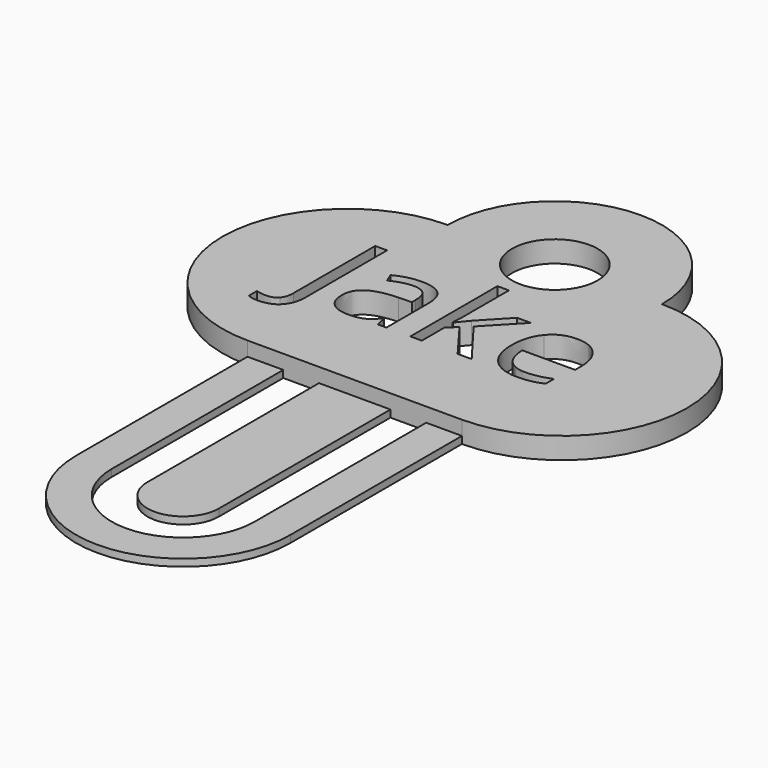
from build123d import *

# Parameters (mm, degrees)
F0_R     = 6
F1_DEPTH = 3
F2_DEPTH = 1


with BuildPart() as f1:
    # F0 (on Top) → F1 (new body)
    with BuildSketch(Plane.XY):
        with BuildLine():
            Line((10, -17.5), (15, -17.5))
            ThreePointArc((15, -17.5), (32.5, 0), (15, 17.5))
            ThreePointArc((15, 17.5), (0, 32.5), (-15, 17.5))
            ThreePointArc((-15, 17.5), (-32.5, 0), (-15, -17.5))
            Line((-15, -17.5), (-10, -17.5))
            Line((-10, -17.5), (-5, -17.5))
            Line((-5, -17.5), (5, -17.5))
            Line((5, -17.5), (10, -17.5))
        make_face()
        with BuildLine():
            add(Edge.make_bspline(
                [(-17.3530564989, -8.385057961), (-18.2929470593, -9.4079721875), (-20.0568083443, -9.4079721875)],
                knots=[0, 0, 0, 1, 1, 1], degree=2))
            add(Edge.make_bspline(
                [(-20.0568083443, -9.4079721875), (-20.974768125, -9.4079721875), (-21.5042398074, -9.1448028306)],
                knots=[0, 0, 0, 1, 1, 1], degree=2))
            Line((-21.5042398074, -9.1448028306), (-21.5042398074, -7.7255680844))
            add(Edge.make_bspline(
                [(-21.5042398074, -7.7255680844), (-20.8087207927, -7.9198121336), (-20.0568083443, -7.9198121336)],
                knots=[0, 0, 0, 1, 1, 1], degree=2))
            add(Edge.make_bspline(
                [(-20.0568083443, -7.9198121336), (-19.0855880986, -7.9198121336), (-18.5811801645, -7.3323805333)],
                knots=[0, 0, 0, 1, 1, 1], degree=2))
            add(Edge.make_bspline(
                [(-18.5811801645, -7.3323805333), (-18.0767722304, -6.7449489331), (-18.0767722304, -5.6390110403)],
                knots=[0, 0, 0, 1, 1, 1], degree=2))
            Line((-18.0767722304, -5.6390110403), (-18.0767722304, 8.6755221946))
            Line((-18.0767722304, 8.6755221946), (-16.4131659385, 8.6755221946))
            Line((-16.4131659385, 8.6755221946), (-16.4131659385, -5.5011604248))
            add(Edge.make_bspline(
                [(-16.4131659385, -5.5011604248), (-16.4131659385, -7.3621437344), (-17.3530564989, -8.385057961)],
                knots=[0, 0, 0, 1, 1, 1], degree=2))
        make_face(mode=Mode.SUBTRACT)
        with BuildLine():
            Line((-5.0561550003, -5.6390110403), (-6.2623478861, -5.6390110403))
            Line((-6.2623478861, -5.6390110403), (-6.5850436452, -4.1101223954))
            Line((-6.5850436452, -4.1101223954), (-6.6633678586, -4.1101223954))
            add(Edge.make_bspline(
                [(-6.6633678586, -4.1101223954), (-7.4654078035, -5.1189382636), (-8.2627482955, -5.4776631608)],
                knots=[0, 0, 0, 1, 1, 1], degree=2))
            add(Edge.make_bspline(
                [(-8.2627482955, -5.4776631608), (-9.0600887876, -5.836388058), (-10.2568827679, -5.836388058)],
                knots=[0, 0, 0, 1, 1, 1], degree=2))
            add(Edge.make_bspline(
                [(-10.2568827679, -5.836388058), (-11.851563752, -5.836388058), (-12.7569916585, -5.0124173334)],
                knots=[0, 0, 0, 1, 1, 1], degree=2))
            add(Edge.make_bspline(
                [(-12.7569916585, -5.0124173334), (-13.6624195651, -4.1884466088), (-13.6624195651, -2.672089838)],
                knots=[0, 0, 0, 1, 1, 1], degree=2))
            add(Edge.make_bspline(
                [(-13.6624195651, -2.672089838), (-13.6624195651, 0.5767985325), (-8.464824766, 0.7334469592)],
                knots=[0, 0, 0, 1, 1, 1], degree=2))
            Line((-8.464824766, 0.7334469592), (-6.6445700474, 0.7929733614))
            Line((-6.6445700474, 0.7929733614), (-6.6445700474, 1.4602956592))
            add(Edge.make_bspline(
                [(-6.6445700474, 1.4602956592), (-6.6445700474, 2.7228819787), (-7.1865736039, 3.3244119374)],
                knots=[0, 0, 0, 1, 1, 1], degree=2))
            add(Edge.make_bspline(
                [(-7.1865736039, 3.3244119374), (-7.7285771604, 3.925941896), (-8.9253711406, 3.925941896)],
                knots=[0, 0, 0, 1, 1, 1], degree=2))
            add(Edge.make_bspline(
                [(-8.9253711406, 3.925941896), (-10.2662816735, 3.925941896), (-11.9580846822, 3.10510414)],
                knots=[0, 0, 0, 1, 1, 1], degree=2))
            Line((-11.9580846822, 3.10510414), (-12.4593596477, 4.3488926482))
            add(Edge.make_bspline(
                [(-12.4593596477, 4.3488926482), (-11.6667186085, 4.7781093375), (-10.7221285953, 5.0224808832)],
                knots=[0, 0, 0, 1, 1, 1], degree=2))
            add(Edge.make_bspline(
                [(-10.7221285953, 5.0224808832), (-9.7775385821, 5.2668524289), (-8.8251161475, 5.2668524289)],
                knots=[0, 0, 0, 1, 1, 1], degree=2))
            add(Edge.make_bspline(
                [(-8.8251161475, 5.2668524289), (-6.9077394043, 5.2668524289), (-5.9819472023, 4.4162514717)],
                knots=[0, 0, 0, 1, 1, 1], degree=2))
            add(Edge.make_bspline(
                [(-5.9819472023, 4.4162514717), (-5.0561550003, 3.5656505146), (-5.0561550003, 1.6858693937)],
                knots=[0, 0, 0, 1, 1, 1], degree=2))
            Line((-5.0561550003, 1.6858693937), (-5.0561550003, -5.6390110403))
        make_face(mode=Mode.SUBTRACT)
        with BuildLine():
            Line((-0.1812559603, -0.146917199), (-0.102931747, -0.146917199))
            add(Edge.make_bspline(
                [(-0.102931747, -0.146917199), (0.3168860367, 0.4514797911), (1.1784523837, 1.4195670683)],
                knots=[0, 0, 0, 1, 1, 1], degree=2))
            Line((1.1784523837, 1.4195670683), (4.6435155831, 5.0914061909))
            Line((4.6435155831, 5.0914061909), (6.5734242004, 5.0914061909))
            Line((6.5734242004, 5.0914061909), (2.2248638743, 0.5204050988))
            Line((2.2248638743, 0.5204050988), (6.8773221483, -5.6390110403))
            Line((6.8773221483, -5.6390110403), (4.9098179085, -5.6390110403))
            Line((4.9098179085, -5.6390110403), (1.1189259815, -0.5667349827))
            Line((1.1189259815, -0.5667349827), (-0.102931747, -1.6256783474))
            Line((-0.102931747, -1.6256783474), (-0.102931747, -5.6390110403))
            Line((-0.102931747, -5.6390110403), (-1.7101446053, -5.6390110403))
            Line((-1.7101446053, -5.6390110403), (-1.7101446053, 9.5966149438))
            Line((-1.7101446053, 9.5966149438), (-0.102931747, 9.5966149438))
            Line((-0.102931747, 9.5966149438), (-0.102931747, 1.5166890929))
            add(Edge.make_bspline(
                [(-0.102931747, 1.5166890929), (-0.102931747, 0.9809514734), (-0.1812559603, -0.146917199)],
                knots=[0, 0, 0, 1, 1, 1], degree=2))
        make_face(mode=Mode.SUBTRACT)
        with BuildLine():
            add(Edge.make_bspline(
                [(15.2016195449, -5.6734736942), (14.4340422539, -5.836388058), (13.3469021724, -5.836388058)],
                knots=[0, 0, 0, 1, 1, 1], degree=2))
            add(Edge.make_bspline(
                [(13.3469021724, -5.836388058), (10.9689790546, -5.836388058), (9.5920393836, -4.3858236265)],
                knots=[0, 0, 0, 1, 1, 1], degree=2))
            add(Edge.make_bspline(
                [(9.5920393836, -4.3858236265), (8.2150997126, -2.9352591949), (8.2150997126, -0.3630920279)],
                knots=[0, 0, 0, 1, 1, 1], degree=2))
            add(Edge.make_bspline(
                [(8.2150997126, -0.3630920279), (8.2150997126, 2.2341388873), (9.4933508747, 3.761461048)],
                knots=[0, 0, 0, 1, 1, 1], degree=2))
            add(Edge.make_bspline(
                [(9.4933508747, 3.761461048), (10.7716020369, 5.2887832086), (12.9270843887, 5.2887832086)],
                knots=[0, 0, 0, 1, 1, 1], degree=2))
            add(Edge.make_bspline(
                [(12.9270843887, 5.2887832086), (14.9415831565, 5.2887832086), (16.116446357, 3.9619710342)],
                knots=[0, 0, 0, 1, 1, 1], degree=2))
            add(Edge.make_bspline(
                [(16.116446357, 3.9619710342), (17.2913095575, 2.6351588598), (17.2913095575, 0.4608786967)],
                knots=[0, 0, 0, 1, 1, 1], degree=2))
            Line((17.2913095575, 0.4608786967), (17.2913095575, -0.5667349827))
            Line((17.2913095575, -0.5667349827), (9.9006367842, -0.5667349827))
            add(Edge.make_bspline(
                [(9.9006367842, -0.5667349827), (9.9507642808, -2.4559150091), (10.8561921873, -3.4349676762)],
                knots=[0, 0, 0, 1, 1, 1], degree=2))
            add(Edge.make_bspline(
                [(10.8561921873, -3.4349676762), (11.7616200938, -4.4140203433), (13.4064285746, -4.4140203433)],
                knots=[0, 0, 0, 1, 1, 1], degree=2))
            add(Edge.make_bspline(
                [(13.4064285746, -4.4140203433), (15.1389601742, -4.4140203433), (16.830763183, -3.6903046118)],
                knots=[0, 0, 0, 1, 1, 1], degree=2))
            Line((16.830763183, -3.6903046118), (16.830763183, -5.1408690433))
            add(Edge.make_bspline(
                [(16.830763183, -5.1408690433), (15.9691968359, -5.5105593304), (15.2016195449, -5.6734736942)],
                knots=[0, 0, 0, 1, 1, 1], degree=2))
        make_face(mode=Mode.SUBTRACT)
        with Locations((0, 17.5)):
            Circle(F0_R, mode=Mode.SUBTRACT)
    extrude(amount=F1_DEPTH)

    # F0 (on Top) → F2 (join)
    with BuildSketch(Plane.XY):
        with BuildLine():
            Line((15, -47.5), (15, -17.5))
            Line((15, -17.5), (10, -17.5))
            Line((10, -17.5), (10, -47.5))
            ThreePointArc((10, -47.5), (0, -57.5), (-10, -47.5))
            Line((-10, -47.5), (-10, -17.5))
            Line((-10, -17.5), (-15, -17.5))
            Line((-15, -17.5), (-15, -47.5))
            ThreePointArc((-15, -47.5), (0, -62.5), (15, -47.5))
        make_face()
        with BuildLine():
            Line((10, -17.5), (15, -17.5))
            ThreePointArc((15, -17.5), (32.5, 0), (15, 17.5))
            ThreePointArc((15, 17.5), (0, 32.5), (-15, 17.5))
            ThreePointArc((-15, 17.5), (-32.5, 0), (-15, -17.5))
            Line((-15, -17.5), (-10, -17.5))
            Line((-10, -17.5), (-5, -17.5))
            Line((-5, -17.5), (5, -17.5))
            Line((5, -17.5), (10, -17.5))
        make_face()
        with BuildLine():
            add(Edge.make_bspline(
                [(-17.3530564989, -8.385057961), (-18.2929470593, -9.4079721875), (-20.0568083443, -9.4079721875)],
                knots=[0, 0, 0, 1, 1, 1], degree=2))
            add(Edge.make_bspline(
                [(-20.0568083443, -9.4079721875), (-20.974768125, -9.4079721875), (-21.5042398074, -9.1448028306)],
                knots=[0, 0, 0, 1, 1, 1], degree=2))
            Line((-21.5042398074, -9.1448028306), (-21.5042398074, -7.7255680844))
            add(Edge.make_bspline(
                [(-21.5042398074, -7.7255680844), (-20.8087207927, -7.9198121336), (-20.0568083443, -7.9198121336)],
                knots=[0, 0, 0, 1, 1, 1], degree=2))
            add(Edge.make_bspline(
                [(-20.0568083443, -7.9198121336), (-19.0855880986, -7.9198121336), (-18.5811801645, -7.3323805333)],
                knots=[0, 0, 0, 1, 1, 1], degree=2))
            add(Edge.make_bspline(
                [(-18.5811801645, -7.3323805333), (-18.0767722304, -6.7449489331), (-18.0767722304, -5.6390110403)],
                knots=[0, 0, 0, 1, 1, 1], degree=2))
            Line((-18.0767722304, -5.6390110403), (-18.0767722304, 8.6755221946))
            Line((-18.0767722304, 8.6755221946), (-16.4131659385, 8.6755221946))
            Line((-16.4131659385, 8.6755221946), (-16.4131659385, -5.5011604248))
            add(Edge.make_bspline(
                [(-16.4131659385, -5.5011604248), (-16.4131659385, -7.3621437344), (-17.3530564989, -8.385057961)],
                knots=[0, 0, 0, 1, 1, 1], degree=2))
        make_face(mode=Mode.SUBTRACT)
        with BuildLine():
            Line((-5.0561550003, -5.6390110403), (-6.2623478861, -5.6390110403))
            Line((-6.2623478861, -5.6390110403), (-6.5850436452, -4.1101223954))
            Line((-6.5850436452, -4.1101223954), (-6.6633678586, -4.1101223954))
            add(Edge.make_bspline(
                [(-6.6633678586, -4.1101223954), (-7.4654078035, -5.1189382636), (-8.2627482955, -5.4776631608)],
                knots=[0, 0, 0, 1, 1, 1], degree=2))
            add(Edge.make_bspline(
                [(-8.2627482955, -5.4776631608), (-9.0600887876, -5.836388058), (-10.2568827679, -5.836388058)],
                knots=[0, 0, 0, 1, 1, 1], degree=2))
            add(Edge.make_bspline(
                [(-10.2568827679, -5.836388058), (-11.851563752, -5.836388058), (-12.7569916585, -5.0124173334)],
                knots=[0, 0, 0, 1, 1, 1], degree=2))
            add(Edge.make_bspline(
                [(-12.7569916585, -5.0124173334), (-13.6624195651, -4.1884466088), (-13.6624195651, -2.672089838)],
                knots=[0, 0, 0, 1, 1, 1], degree=2))
            add(Edge.make_bspline(
                [(-13.6624195651, -2.672089838), (-13.6624195651, 0.5767985325), (-8.464824766, 0.7334469592)],
                knots=[0, 0, 0, 1, 1, 1], degree=2))
            Line((-8.464824766, 0.7334469592), (-6.6445700474, 0.7929733614))
            Line((-6.6445700474, 0.7929733614), (-6.6445700474, 1.4602956592))
            add(Edge.make_bspline(
                [(-6.6445700474, 1.4602956592), (-6.6445700474, 2.7228819787), (-7.1865736039, 3.3244119374)],
                knots=[0, 0, 0, 1, 1, 1], degree=2))
            add(Edge.make_bspline(
                [(-7.1865736039, 3.3244119374), (-7.7285771604, 3.925941896), (-8.9253711406, 3.925941896)],
                knots=[0, 0, 0, 1, 1, 1], degree=2))
            add(Edge.make_bspline(
                [(-8.9253711406, 3.925941896), (-10.2662816735, 3.925941896), (-11.9580846822, 3.10510414)],
                knots=[0, 0, 0, 1, 1, 1], degree=2))
            Line((-11.9580846822, 3.10510414), (-12.4593596477, 4.3488926482))
            add(Edge.make_bspline(
                [(-12.4593596477, 4.3488926482), (-11.6667186085, 4.7781093375), (-10.7221285953, 5.0224808832)],
                knots=[0, 0, 0, 1, 1, 1], degree=2))
            add(Edge.make_bspline(
                [(-10.7221285953, 5.0224808832), (-9.7775385821, 5.2668524289), (-8.8251161475, 5.2668524289)],
                knots=[0, 0, 0, 1, 1, 1], degree=2))
            add(Edge.make_bspline(
                [(-8.8251161475, 5.2668524289), (-6.9077394043, 5.2668524289), (-5.9819472023, 4.4162514717)],
                knots=[0, 0, 0, 1, 1, 1], degree=2))
            add(Edge.make_bspline(
                [(-5.9819472023, 4.4162514717), (-5.0561550003, 3.5656505146), (-5.0561550003, 1.6858693937)],
                knots=[0, 0, 0, 1, 1, 1], degree=2))
            Line((-5.0561550003, 1.6858693937), (-5.0561550003, -5.6390110403))
        make_face(mode=Mode.SUBTRACT)
        with BuildLine():
            Line((-0.1812559603, -0.146917199), (-0.102931747, -0.146917199))
            add(Edge.make_bspline(
                [(-0.102931747, -0.146917199), (0.3168860367, 0.4514797911), (1.1784523837, 1.4195670683)],
                knots=[0, 0, 0, 1, 1, 1], degree=2))
            Line((1.1784523837, 1.4195670683), (4.6435155831, 5.0914061909))
            Line((4.6435155831, 5.0914061909), (6.5734242004, 5.0914061909))
            Line((6.5734242004, 5.0914061909), (2.2248638743, 0.5204050988))
            Line((2.2248638743, 0.5204050988), (6.8773221483, -5.6390110403))
            Line((6.8773221483, -5.6390110403), (4.9098179085, -5.6390110403))
            Line((4.9098179085, -5.6390110403), (1.1189259815, -0.5667349827))
            Line((1.1189259815, -0.5667349827), (-0.102931747, -1.6256783474))
            Line((-0.102931747, -1.6256783474), (-0.102931747, -5.6390110403))
            Line((-0.102931747, -5.6390110403), (-1.7101446053, -5.6390110403))
            Line((-1.7101446053, -5.6390110403), (-1.7101446053, 9.5966149438))
            Line((-1.7101446053, 9.5966149438), (-0.102931747, 9.5966149438))
            Line((-0.102931747, 9.5966149438), (-0.102931747, 1.5166890929))
            add(Edge.make_bspline(
                [(-0.102931747, 1.5166890929), (-0.102931747, 0.9809514734), (-0.1812559603, -0.146917199)],
                knots=[0, 0, 0, 1, 1, 1], degree=2))
        make_face(mode=Mode.SUBTRACT)
        with BuildLine():
            add(Edge.make_bspline(
                [(15.2016195449, -5.6734736942), (14.4340422539, -5.836388058), (13.3469021724, -5.836388058)],
                knots=[0, 0, 0, 1, 1, 1], degree=2))
            add(Edge.make_bspline(
                [(13.3469021724, -5.836388058), (10.9689790546, -5.836388058), (9.5920393836, -4.3858236265)],
                knots=[0, 0, 0, 1, 1, 1], degree=2))
            add(Edge.make_bspline(
                [(9.5920393836, -4.3858236265), (8.2150997126, -2.9352591949), (8.2150997126, -0.3630920279)],
                knots=[0, 0, 0, 1, 1, 1], degree=2))
            add(Edge.make_bspline(
                [(8.2150997126, -0.3630920279), (8.2150997126, 2.2341388873), (9.4933508747, 3.761461048)],
                knots=[0, 0, 0, 1, 1, 1], degree=2))
            add(Edge.make_bspline(
                [(9.4933508747, 3.761461048), (10.7716020369, 5.2887832086), (12.9270843887, 5.2887832086)],
                knots=[0, 0, 0, 1, 1, 1], degree=2))
            add(Edge.make_bspline(
                [(12.9270843887, 5.2887832086), (14.9415831565, 5.2887832086), (16.116446357, 3.9619710342)],
                knots=[0, 0, 0, 1, 1, 1], degree=2))
            add(Edge.make_bspline(
                [(16.116446357, 3.9619710342), (17.2913095575, 2.6351588598), (17.2913095575, 0.4608786967)],
                knots=[0, 0, 0, 1, 1, 1], degree=2))
            Line((17.2913095575, 0.4608786967), (17.2913095575, -0.5667349827))
            Line((17.2913095575, -0.5667349827), (9.9006367842, -0.5667349827))
            add(Edge.make_bspline(
                [(9.9006367842, -0.5667349827), (9.9507642808, -2.4559150091), (10.8561921873, -3.4349676762)],
                knots=[0, 0, 0, 1, 1, 1], degree=2))
            add(Edge.make_bspline(
                [(10.8561921873, -3.4349676762), (11.7616200938, -4.4140203433), (13.4064285746, -4.4140203433)],
                knots=[0, 0, 0, 1, 1, 1], degree=2))
            add(Edge.make_bspline(
                [(13.4064285746, -4.4140203433), (15.1389601742, -4.4140203433), (16.830763183, -3.6903046118)],
                knots=[0, 0, 0, 1, 1, 1], degree=2))
            Line((16.830763183, -3.6903046118), (16.830763183, -5.1408690433))
            add(Edge.make_bspline(
                [(16.830763183, -5.1408690433), (15.9691968359, -5.5105593304), (15.2016195449, -5.6734736942)],
                knots=[0, 0, 0, 1, 1, 1], degree=2))
        make_face(mode=Mode.SUBTRACT)
        with Locations((0, 17.5)):
            Circle(F0_R, mode=Mode.SUBTRACT)
        with BuildLine():
            Line((5, -47.5), (5, -17.5))
            Line((5, -17.5), (-5, -17.5))
            Line((-5, -17.5), (-5, -47.5))
            ThreePointArc((-5, -47.5), (0, -52.5), (5, -47.5))
        make_face()
    extrude(amount=F2_DEPTH)


solid = f1.part
